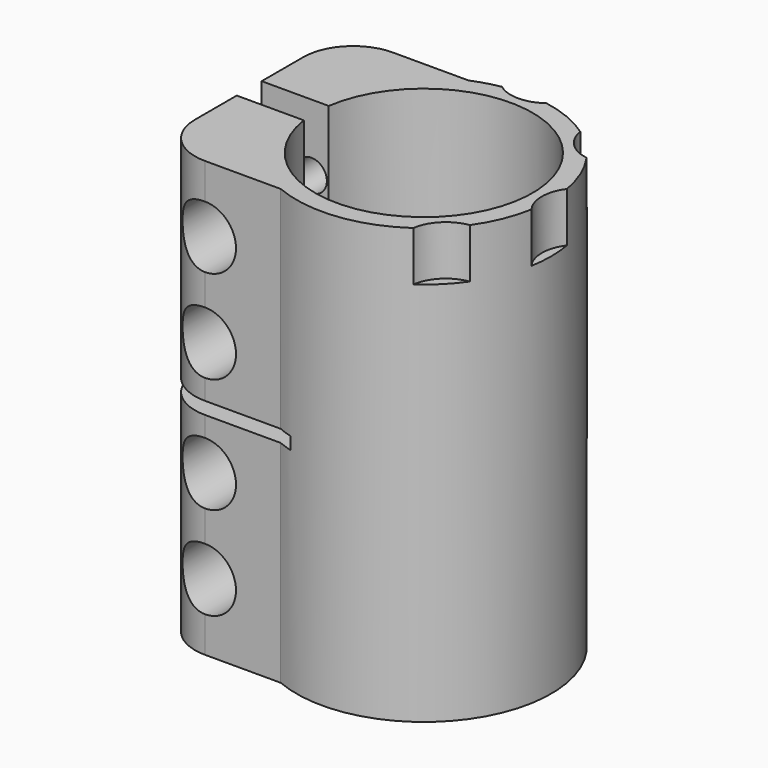
from build123d import *

# Parameters (mm, degrees)
F1_DEPTH       = 35
F3_D           = 5
F3_START       = 1.7550021
F3_CBORE_D     = 10
F3_CBORE_DEPTH = 8
F4_W           = 22.4
F4_H           = 2
F5_DEPTH       = 25
F7_DEPTH       = 8


with BuildPart() as f1:
    # F0 (on Top) → F1 (new body, symmetric)
    with BuildSketch(Plane.XY):
        with BuildLine():
            ThreePointArc((-17.3192642082, 2.5086026559), (17.5, 0), (-17.3192642082, -2.5086026559))
            Line((-17.3192642082, -2.5086026559), (-28.1192642082, -2.5086026559))
            Line((-28.1192642082, -2.5086026559), (-28.1192642082, -10.9086026559))
            ThreePointArc((-28.1192642082, -10.9086026559), (-25.7761184577, -16.5654569054), (-20.1192642082, -18.9086026559))
            Line((-20.1192642082, -18.9086026559), (-7.9192642082, -18.9086026559))
            ThreePointArc((-7.9192642082, -18.9086026559), (20.5, 0), (-7.9192642082, 18.9086026559))
            Line((-7.9192642082, 18.9086026559), (-20.1192642082, 18.9086026559))
            ThreePointArc((-20.1192642082, 18.9086026559), (-25.7761184577, 16.5654569054), (-28.1192642082, 10.9086026559))
            Line((-28.1192642082, 10.9086026559), (-28.1192642082, 2.5086026559))
            Line((-28.1192642082, 2.5086026559), (-17.3192642082, 2.5086026559))
        make_face()
    extrude(amount=F1_DEPTH, both=True)

    # F3 (through all)
    # its depths count from where the whole tool has entered the part; down to there all is cleared
    with Locations(Plane.XZ.offset(18.9086026559).offset(-F3_START)):
        with Locations((-20.1192642082, 24.25), (-20.1192642082, 9.25), (-20.1192642082, -9.25), (-20.1192642082, -24.25)):
            CounterBoreHole(F3_D / 2, F3_CBORE_D / 2, F3_CBORE_DEPTH)

    # F4 (on Front) → F5 (cut, symmetric)
    with BuildSketch(Plane.XZ):
        with Locations((-16.9192642082, 0)):
            Rectangle(F4_W, F4_H)
    extrude(amount=F5_DEPTH, both=True, mode=Mode.SUBTRACT)

    # F6 (on face) → F7 (cut)
    with BuildSketch(Plane.XY.offset(35)):
        with BuildLine():
            ThreePointArc((16.8043309304, -11.7415698261), (14.4956890143, -14.4956890143), (11.7415698261, -16.8043309304))
            ThreePointArc((11.7415698261, -16.8043309304), (17.2398329286, -23.6616731318), (23.6776695297, -17.6776695297))
            ThreePointArc((23.6776695297, -17.6776695297), (21.5994018258, -13.1367427743), (16.8043309304, -11.7415698261))
        make_face()
        with BuildLine():
            ThreePointArc((16.8043309304, -11.7415698261), (13.4350288425, -13.4350288425), (11.7415698261, -16.8043309304))
            ThreePointArc((11.7415698261, -16.8043309304), (14.4956890143, -14.4956890143), (16.8043309304, -11.7415698261))
        make_face()
        with BuildLine():
            ThreePointArc((20.185, 3.5799127084), (20.5, 0), (20.185, -3.5799127084))
            ThreePointArc((20.185, -3.5799127084), (26.8854707635, -5.6960512638), (31, 0))
            ThreePointArc((31, 0), (26.8854707635, 5.6960512638), (20.185, 3.5799127084))
        make_face()
        with BuildLine():
            ThreePointArc((20.185, 3.5799127084), (19, 0), (20.185, -3.5799127084))
            ThreePointArc((20.185, -3.5799127084), (20.5, 0), (20.185, 3.5799127084))
        make_face()
        with BuildLine():
            ThreePointArc((11.7415698261, 16.8043309304), (14.4956890143, 14.4956890143), (16.8043309304, 11.7415698261))
            ThreePointArc((16.8043309304, 11.7415698261), (21.5994018258, 13.1367427743), (23.6776695297, 17.6776695297))
            ThreePointArc((23.6776695297, 17.6776695297), (17.2398329286, 23.6616731318), (11.7415698261, 16.8043309304))
        make_face()
        with BuildLine():
            ThreePointArc((11.7415698261, 16.8043309304), (13.4350288425, 13.4350288425), (16.8043309304, 11.7415698261))
            ThreePointArc((16.8043309304, 11.7415698261), (14.4956890143, 14.4956890143), (11.7415698261, 16.8043309304))
        make_face()
        with BuildLine():
            ThreePointArc((-3.5799127084, 20.185), (0, 20.5), (3.5799127084, 20.185))
            ThreePointArc((3.5799127084, 20.185), (5.3609456372, 22.305512688), (6, 25))
            ThreePointArc((6, 25), (-2.694487312, 30.3609456372), (-3.5799127084, 20.185))
        make_face()
        with BuildLine():
            ThreePointArc((-3.5799127084, 20.185), (0, 19), (3.5799127084, 20.185))
            ThreePointArc((3.5799127084, 20.185), (0, 20.5), (-3.5799127084, 20.185))
        make_face()
    extrude(amount=-F7_DEPTH, mode=Mode.SUBTRACT)


solid = f1.part
